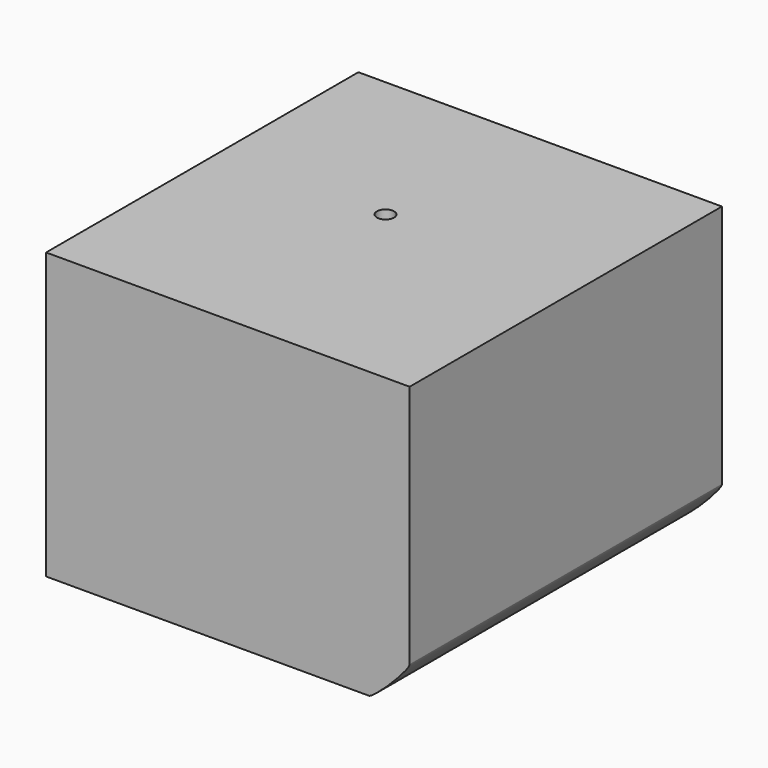
from build123d import *

# Parameters (mm, degrees)
F0_W          = 89.2122089863
F0_H          = 95.7951173186
F1_DEPTH      = 20
F1_DEPTH_BACK = 50
F2_T1_DEPTH   = 145.7951173186
F4_D          = 4.2
F5_W          = 53.7064000964
F5_H          = 35.0269903429
F6_DEPTH      = 10


# Not quite as in the source:
# - a fillet or chamfer that OpenCascade refuses, or shapes differently, is made with other operations: its cross-section is extruded or revolved along the edge and cut away or added


with BuildPart() as f1:
    # F0 (on Top) → F1 (new body, two sides)
    with BuildSketch(Plane.XY) as f1_sk:
        with Locations((44.6061044931, 47.8975586593)):
            Rectangle(F0_W, F0_H)
    extrude(amount=-F1_DEPTH)
    extrude(f1_sk.sketch, amount=F1_DEPTH_BACK)

    # F2: fillet of radius 10 on 1 edges, made by hand

    # F2_s2 → F2_t1 (cut)
    with BuildSketch(Plane.XZ.offset(-120.7951173186)):
        with BuildLine():
            add(Edge.make_bspline(
                [(89.2122089863, -10), (89.2122089863, -20), (79.2122089863, -20)],
                knots=[0, 0, 0, 1, 1, 1], degree=2, weights=[1, 0.1111111111, 1]))
            Line((79.2122089863, -20), (89.2122089863, -20))
            Line((89.2122089863, -20), (89.2122089863, -10))
        make_face()
    extrude(amount=F2_T1_DEPTH, mode=Mode.SUBTRACT)

    # F4 (through all)
    with Locations(Plane(origin=(0, 0, -20), x_dir=(1, 0, 0), z_dir=(0, 0, -1))):
        with Locations((40.9390032291, -52.9426522553)):
            Hole(F4_D / 2)

    # F5 (on face) → F6 (cut)
    with BuildSketch(Plane(origin=(0, 0, -20), x_dir=(1, 0, 0), z_dir=(0, 0, -1))):
        with Locations((43.4090383351, -23.1333931442)):
            Rectangle(F5_W, F5_H)
    extrude(amount=-F6_DEPTH, mode=Mode.SUBTRACT)


solid = f1.part
